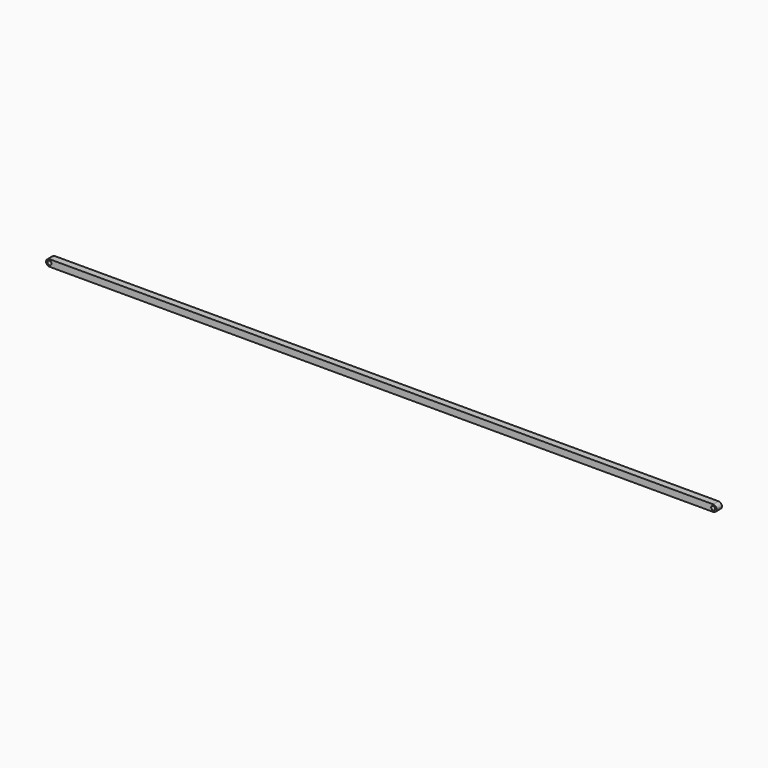
from build123d import *

# Parameters (mm, degrees)
F0_W     = 500
F0_H     = 5
F0_R     = 1.5
F1_DEPTH = 5
F2_R     = 2.49999


# Not quite as in the source:
# - a fillet or chamfer is up to 0.001 mm smaller than in the source, because OpenCascade refuses the exact size


with BuildPart() as f1:
    # F0 (on Front) → F1 (new body)
    with BuildSketch(Plane.XZ):
        Rectangle(F0_W, F0_H)
        with Locations((-247.5, 0)):
            Circle(F0_R, mode=Mode.SUBTRACT)
        with Locations((247.5, 0)):
            Circle(F0_R, mode=Mode.SUBTRACT)
    extrude(amount=F1_DEPTH)

    # F2 (radius 2.5 in the source; OpenCascade refuses exactly that, so slightly less here)
    f2_edges = [f1.edges().sort_by_distance(p)[0] for p in [
        (250, -2.5, 2.5),
        (250, -2.5, -2.5),
        (-250, -2.5, 2.5),
        (-250, -2.5, -2.5),
    ]]
    fillet(f2_edges, radius=F2_R)


solid = f1.part
